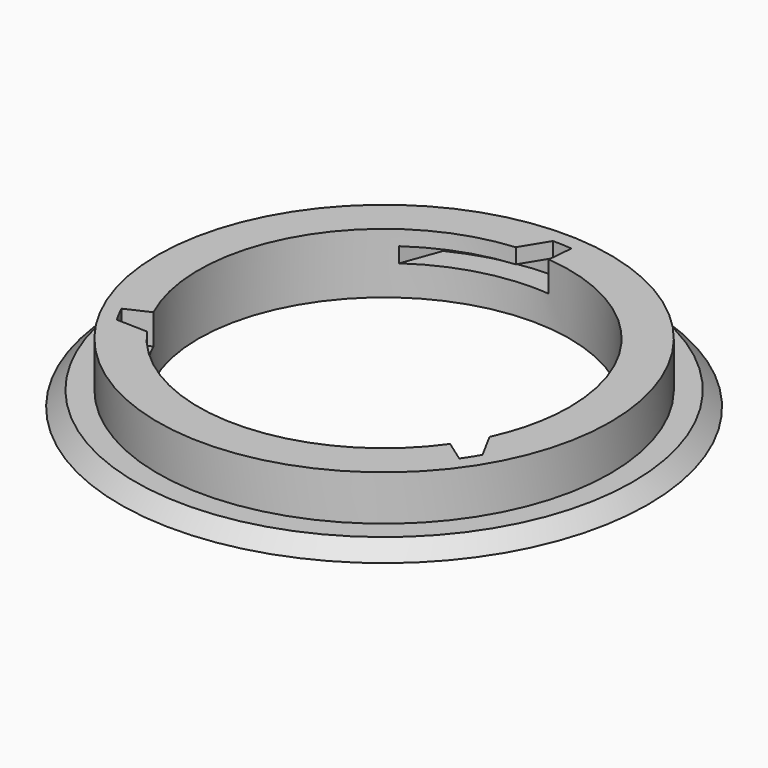
from build123d import *

# Parameters (mm, degrees)
F0_R     = 44.45
F0_R_2   = 31.242
F1_DEPTH = 2.54
F2_R     = 38.1
F2_R_2   = 31.242
F3_DEPTH = 5.08
F5_DEPTH = 2.54
F6_R     = 38.1
F6_R_2   = 31.242
F7_DEPTH = 2.54
F9_DEPTH = 2.54
F10_SIZE = 2.53999


# Not quite as in the source:
# - a fillet or chamfer is up to 0.001 mm smaller than in the source, because OpenCascade refuses the exact size


with BuildPart() as f1:
    # F0 (on Top) → F1 (new body)
    with BuildSketch(Plane.XY):
        Circle(F0_R)
        Circle(F0_R_2, mode=Mode.SUBTRACT)
    extrude(amount=F1_DEPTH)

    # F2 (on face) → F3 (join)
    with BuildSketch(Plane.XY.offset(2.54)):
        Circle(F2_R)
        Circle(F2_R_2, mode=Mode.SUBTRACT)
    extrude(amount=F3_DEPTH)

    # F4 (on face) → F5 (cut)
    with BuildSketch(Plane.XY.offset(7.62)):
        with BuildLine():
            ThreePointArc((-25.5919481677, -17.9196750245), (-27.0835882302, -15.5737539654), (-28.3607839843, -13.1045219598))
            Line((-28.3607839843, -13.1045219598), (-32.2805671366, -14.9157160518))
            ThreePointArc((-32.2805671366, -14.9157160518), (-31.5707150955, -16.3647043469), (-30.7958633586, -17.78))
            ThreePointArc((-30.7958633586, -17.78), (-26.0009342584, -24.2582979142), (-19.8703037457, -29.4904158847))
            Line((-19.8703037457, -29.4904158847), (-13.2034397333, -28.3148678826))
            ThreePointArc((-13.2034397333, -28.3148678826), (-20.0819705018, -23.9327604919), (-25.5919481677, -17.9196750245))
        make_face()
        with BuildLine():
            ThreePointArc((-17.9196750245, 25.5919481677), (-10.6853933178, 29.3578768586), (-2.7229197149, 31.1231147578))
            ThreePointArc((-2.7229197149, 31.1231147578), (0.0545275488, 31.2419524157), (2.8315430705, 31.1134203816))
            Line((2.8315430705, 31.1134203816), (3.2228945518, 35.4136492148))
            ThreePointArc((3.2228945518, 35.4136492148), (1.6131078579, 35.5233934618), (0, 35.56))
            ThreePointArc((0, 35.56), (-8.007835117, 34.646618547), (-15.6042974515, 31.9533957671))
            Line((-15.6042974515, 31.9533957671), (-17.9196750245, 25.5919481677))
        make_face()
        with BuildLine():
            Line((35.4746011972, -2.4629798824), (31.1231147578, 2.7229197149))
            ThreePointArc((31.1231147578, 2.7229197149), (31.2122645387, 1.3627569001), (31.242, 0))
            ThreePointArc((31.242, 0), (29.7795828432, -9.4466401268), (25.5292409138, -18.0088984218))
            Line((25.5292409138, -18.0088984218), (29.0576725848, -20.497933163))
            ThreePointArc((29.0576725848, -20.497933163), (29.9576072376, -19.1586891148), (30.7958633586, -17.78))
            ThreePointArc((30.7958633586, -17.78), (34.0087693754, -10.3883206328), (35.4746011972, -2.4629798824))
        make_face()
    extrude(amount=-F5_DEPTH, mode=Mode.SUBTRACT)

    # F6 (on face) → F7 (join)
    with BuildSketch(Plane.XY.offset(7.62)):
        Circle(F6_R)
        Circle(F6_R_2, mode=Mode.SUBTRACT)
    extrude(amount=F7_DEPTH)

    # F8 (on face) → F9 (cut)
    with BuildSketch(Plane.XY.offset(10.16)):
        with BuildLine():
            ThreePointArc((-25.5919481677, -17.9196750245), (-27.0835882302, -15.5737539654), (-28.3607839843, -13.1045219598))
            Line((-28.3607839843, -13.1045219598), (-32.2805671366, -14.9157160518))
            ThreePointArc((-32.2805671366, -14.9157160518), (-31.5707150955, -16.3647043469), (-30.7958633586, -17.78))
            Line((-30.7958633586, -17.78), (-25.5919481677, -17.9196750245))
        make_face()
        with BuildLine():
            ThreePointArc((28.3148678826, -13.2034397333), (27.0290606814, -15.6681984503), (25.5292409138, -18.0088984218))
            Line((25.5292409138, -18.0088984218), (29.0576725848, -20.497933163))
            ThreePointArc((29.0576725848, -20.497933163), (29.9576072376, -19.1586891148), (30.7958633586, -17.78))
            Line((30.7958633586, -17.78), (28.3148678826, -13.2034397333))
        make_face()
        with BuildLine():
            Line((0, 35.56), (-2.7229197149, 31.1231147578))
            ThreePointArc((-2.7229197149, 31.1231147578), (0.0545275488, 31.2419524157), (2.8315430705, 31.1134203816))
            Line((2.8315430705, 31.1134203816), (3.2228945518, 35.4136492148))
            ThreePointArc((3.2228945518, 35.4136492148), (1.6131078579, 35.5233934618), (0, 35.56))
        make_face()
    extrude(amount=-F9_DEPTH, mode=Mode.SUBTRACT)

    # F10 (size 2.54 in the source; OpenCascade refuses exactly that, so slightly less here)
    f10_edges = [f1.edges().sort_by_distance(p)[0] for p in [
        (-44.45, 0, 2.54),
    ]]
    chamfer(f10_edges, length=F10_SIZE)


solid = f1.part
